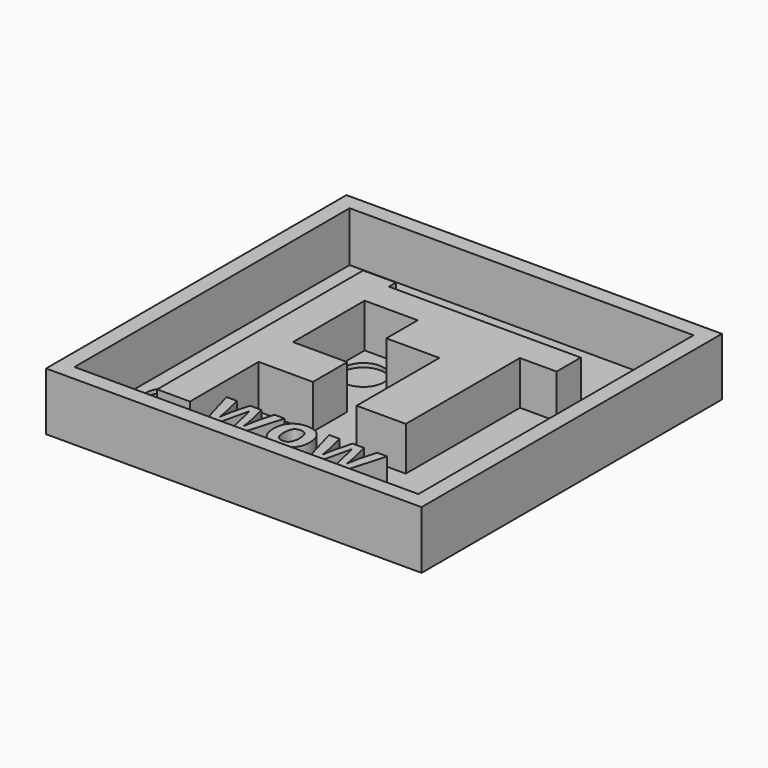
from build123d import *

# Parameters (mm, degrees)
F0_W         = 38.1
F0_H         = 38.1
F1_DEPTH     = 0.79375
F2_W         = 38.1
F2_H         = 38.1
F2_W_2       = 34.8996
F2_H_2       = 34.8996
F3_DEPTH     = 5.08
F5_DEPTH     = 4.445
F4_R         = 2.0516011864
F4_R_2       = 2.0535877667
F6_DEPTH     = 0.396875
F7_TEXT_SIZE = 7.0555555556
F8_DEPTH     = 4.445


# Not quite as in the source:
# - a feature names something its author has since deleted; it is built from what else it names
# - Text() gives the source's letters only with a copy of the font that has no kerning and outlines rounded to 1/6400 em; it was checked with that copy


with BuildPart() as f1:
    # F0 (on Top) → F1 (new body)
    with BuildSketch(Plane.XY):
        with Locations((-0.5674473941, -9.7853171236)):
            Rectangle(F0_W, F0_H)
    extrude(amount=F1_DEPTH)

    # F2 (on face) → F3 (join)
    with BuildSketch(Plane.XY.offset(0.79375)):
        with Locations((-0.5674473941, -9.7853171236)):
            Rectangle(F2_W, F2_H)
        with Locations((-0.5674473941, -9.7853171236)):
            Rectangle(F2_W_2, F2_H_2, mode=Mode.SUBTRACT)
    extrude(amount=F3_DEPTH)

    # F4 (on face) → F5 (join)
    with BuildSketch(Plane.XY.offset(0.79375)):
        Polygon((-7.9350350425, 0.9419018752), (-11.265616864, 0.9419018752), (-11.265616864, -25.1903608441), (-7.9350350425, -25.1903608441), (-7.9350350425, -16.4796076715), (-2.4267639965, -16.4796076715), (-2.4267639965, -12.1242294845), (-7.9350350425, -12.1242294845), (-7.9350350425, -3.0291776638), (-2.5548629928, -3.0291776638), (-2.5548629928, -7.0002567954), (2.8253090568, -7.0002567954), (2.8253090568, -17.504401505), (7.8211827204, -17.504401505), (7.8211827204, -3.0291776638), (11.5360636264, -3.0291776638), (11.5360636264, 0.0452065215), (-7.9350350425, 0.0452065215), align=None)
    extrude(amount=F5_DEPTH)

    # F4 (on face) → F6 (cut)
    with BuildSketch(Plane.XY.offset(0.79375)):
        with Locations((-14.8769598454, -19.5560026914)):
            Circle(F4_R)
        with Locations((-5.3857392631, -6.3803032972)):
            Circle(F4_R_2)
    extrude(amount=-F6_DEPTH, mode=Mode.SUBTRACT)

    # F7 (on face) → F8 (join)
    with BuildSketch(Plane.XY.offset(0.79375)):
        with Locations((-6.2229394822, -26.6320739787)):
            Text('wow', F7_TEXT_SIZE, font='Open Sans', font_style=FontStyle.BOLD, text_align=(TextAlign.LEFT, TextAlign.BOTTOM))
    extrude(amount=F8_DEPTH)


solid = f1.part
